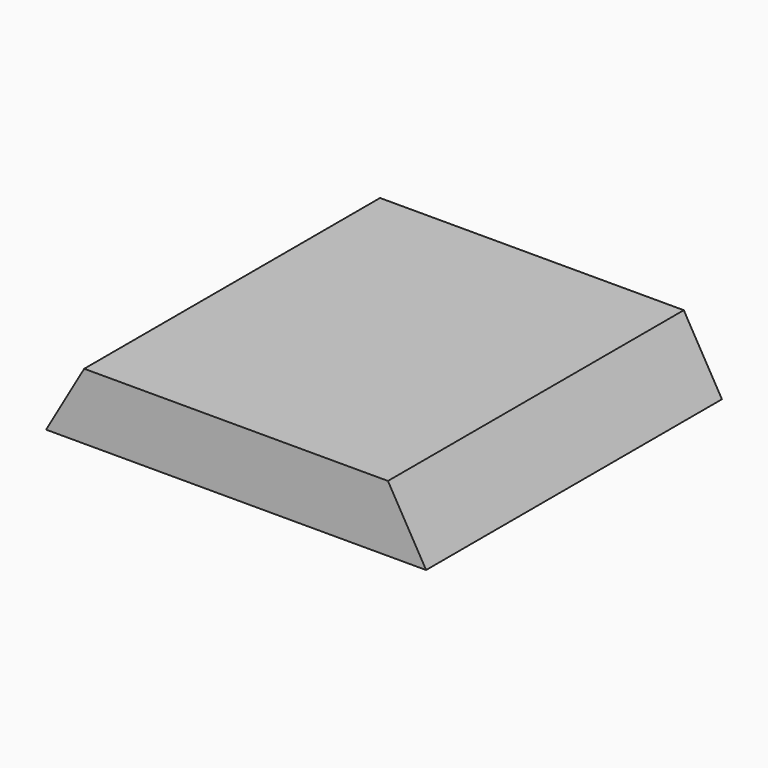
from build123d import *

# Parameters (mm, degrees)
F0_W        = 46.0375
F0_H        = 44.45
F1_DEPTH    = 7.9375
F2_T1_DEPTH = 87.1311818198


# Not quite as in the source:
# - a fillet or chamfer that OpenCascade refuses, or shapes differently, is made with other operations: its cross-section is extruded or revolved along the edge and cut away or added


with BuildPart() as f1:
    # F0 (on Top) → F1 (new body)
    with BuildSketch(Plane.XY):
        with Locations((3.8099996746, 17.1172746531)):
            Rectangle(F0_W, F0_H)
    extrude(amount=F1_DEPTH)

    # F2: chamfer of 4.7625 x 8.248891971 on 2 edges, made by hand

    # F2_s2 → F2_t1 (cut)
    with BuildSketch(Plane.XZ.offset(-60.682865563)):
        Polygon((-19.2087503254, -0.311391971), (-14.4462503254, 7.9375), (-19.2087503254, 7.9375), align=None)
        Polygon((26.8287496746, -0.311391971), (22.0662496746, 7.9375), (26.8287496746, 7.9375), align=None)
    extrude(amount=F2_T1_DEPTH, mode=Mode.SUBTRACT)


solid = f1.part
